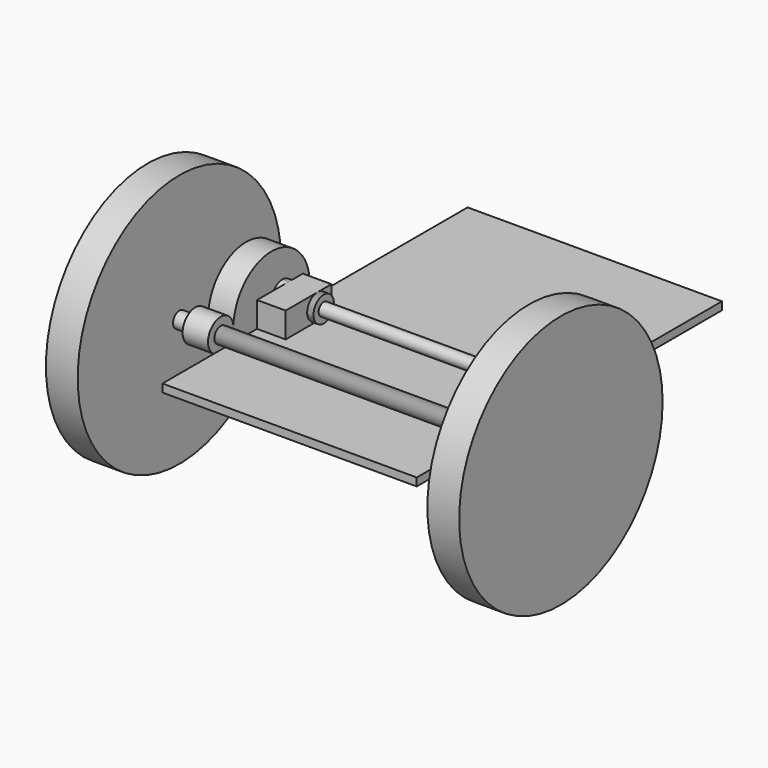
from build123d import *

# Parameters (mm, degrees)
F0_W      = 101.6
F0_H      = 152.4
F1_DEPTH  = 3.175
F3_DEPTH  = 114.3
F4_DEPTH  = 12.7
F5_R      = 6.35
F5_R_2    = 3.175
F6_DEPTH  = 10.16
F7_R      = 3.175
F8_DEPTH  = 6.35
F10_DEPTH = 16.51
F11_W     = 11.43
F11_H     = 22.86
F12_DEPTH = 10.16
F14_DEPTH = 2.54
F15_R     = 2.54
F16_DEPTH = 73.66
F17_DEPTH = 3.81
F18_R     = 5.08
F18_R_2   = 2.54
F19_DEPTH = 2.54
F20_DEPTH = 16.51
F21_DEPTH = 2.54
F22_R     = 50.8
F23_DEPTH = 12.7
F25_DEPTH = 2.54


with BuildPart() as f1:
    # F0 (on Top) → F1 (new body)
    with BuildSketch(Plane.XY):
        Rectangle(F0_W, F0_H)
    extrude(amount=F1_DEPTH)


with BuildPart() as f3:
    # F2 (on face) → F3 (new body)
    with BuildSketch(Plane.YZ.offset(50.8)):
        with BuildLine():
            ThreePointArc((-43.9096465707, 3.175), (-41.6645825404, 4.1049359697), (-40.7346465707, 6.35))
            ThreePointArc((-40.7346465707, 6.35), (-46.1547106009, 8.5950640303), (-43.9096465707, 3.175))
        make_face()
    extrude(amount=-F3_DEPTH)

    # F4 (add): a face of the model
    f4_faces = [f3.faces().sort_by_distance(p)[0] for p in [
        (50.8, -43.9096465707, 6.35),
    ]]
    extrude(f4_faces, amount=F4_DEPTH)

    # F5 (on face) → F6 (join)
    with BuildSketch(Plane.YZ.offset(63.5)):
        with Locations((-43.9096465707, 6.35)):
            Circle(F5_R)
        with Locations((-43.9096465707, 6.35)):
            Circle(F5_R_2, mode=Mode.SUBTRACT)
    extrude(amount=-F6_DEPTH)

    # F7 (on face) → F8 (join)
    with BuildSketch(Plane.YZ.offset(63.5)):
        with Locations((-43.9096465707, 6.35)):
            Circle(F7_R)
    extrude(amount=F8_DEPTH)

    # F22 (on face) → F23 (join)
    with BuildSketch(Plane.YZ.offset(69.85)):
        with Locations((-43.9096465707, 6.35)):
            Circle(F22_R)
    extrude(amount=F23_DEPTH)


with BuildPart() as f10:
    # F9 (on face) → F10 (new body)
    with BuildSketch(Plane.YZ.offset(69.85)):
        with BuildLine():
            ThreePointArc((0.5403534293, 6.35), (-18.5096465707, 25.4), (-37.5596465707, 6.35))
            ThreePointArc((-37.5596465707, 6.35), (-18.5096465707, -12.7), (0.5403534293, 6.35))
        make_face()
    extrude(amount=-F10_DEPTH)

    # F17 (cut): a face of the model
    f17_faces = [f10.faces().sort_by_distance(p)[0] for p in [
        (69.85, -18.5096465707, 6.35),
    ]]
    extrude(f17_faces, amount=-F17_DEPTH, mode=Mode.SUBTRACT)

    # F21 (cut): a face of the model
    f21_faces = [f10.faces().sort_by_distance(p)[0] for p in [
        (66.04, -18.5096465707, 6.35),
    ]]
    extrude(f21_faces, amount=-F21_DEPTH, mode=Mode.SUBTRACT)


with BuildPart() as f12:
    # F11 (on face) → F12 (new body)
    with BuildSketch(Plane.XY.offset(3.175)):
        with Locations((45.085, -17.5209892464)):
            Rectangle(F11_W, F11_H)
    extrude(amount=F12_DEPTH)


with BuildPart() as f14:
    # F13 (on face) → F14 (new body)
    with BuildSketch(Plane(origin=(39.37, 0, 0), x_dir=(0, -1, 0), z_dir=(-1, 0, 0))):
        with BuildLine():
            ThreePointArc((13.1286922842, 3.175), (16.7207947327, 4.6628975516), (18.2086922842, 8.255))
            ThreePointArc((18.2086922842, 8.255), (16.7207947327, 11.8471024484), (13.1286922842, 13.335))
            ThreePointArc((13.1286922842, 13.335), (8.0486922842, 8.255), (13.1286922842, 3.175))
        make_face()
    extrude(amount=F14_DEPTH)


with BuildPart() as f16:
    # F15 (on face) → F16 (new body)
    with BuildSketch(Plane(origin=(36.83, 0, 0), x_dir=(0, -1, 0), z_dir=(-1, 0, 0))):
        with Locations((13.1286922842, 8.255)):
            Circle(F15_R)
    extrude(amount=F16_DEPTH)


with BuildPart() as f19:
    # F18 (on face) → F19 (new body)
    with BuildSketch(Plane(origin=(-36.83, 0, 0), x_dir=(0, -1, 0), z_dir=(-1, 0, 0))):
        with Locations((13.1286922842, 8.255)):
            Circle(F18_R)
        with Locations((13.1286922842, 8.255)):
            Circle(F18_R_2, mode=Mode.SUBTRACT)
    extrude(amount=F19_DEPTH)


with BuildPart() as f20:
    # F20 (new): a face of the model
    f20_faces = [f14.part.faces().sort_by_distance(p)[0] for p in [
        (36.83, -13.1286922842, 8.255),
    ]]
    extrude(f20_faces, amount=-F20_DEPTH)


with BuildPart() as f25:
    # F25 (new): a face of the model
    f25_faces = [f16.part.faces().sort_by_distance(p)[0] for p in [
        (-36.83, -13.1286922842, 8.255),
    ]]
    extrude(f25_faces, amount=F25_DEPTH)


with BuildPart() as f29_1:
    # F29: instance of F3
    add(f3.part.mirror(Plane(origin=(0, 76.2, 3.175), x_dir=(0, -0.9991330731, -0.0416305447), z_dir=(1, 0, 0))))


with BuildPart() as f29_2:
    # F29: instance of F10
    add(f10.part.mirror(Plane(origin=(0, 76.2, 3.175), x_dir=(0, -0.9991330731, -0.0416305447), z_dir=(1, 0, 0))))


with BuildPart() as f29_3:
    # F29: instance of F12
    add(f12.part.mirror(Plane(origin=(0, 76.2, 3.175), x_dir=(0, -0.9991330731, -0.0416305447), z_dir=(1, 0, 0))))


with BuildPart() as f29_4:
    # F29: instance of F14
    add(f14.part.mirror(Plane(origin=(0, 76.2, 3.175), x_dir=(0, -0.9991330731, -0.0416305447), z_dir=(1, 0, 0))))


with BuildPart() as f29_5:
    # F29: instance of F16
    add(f16.part.mirror(Plane(origin=(0, 76.2, 3.175), x_dir=(0, -0.9991330731, -0.0416305447), z_dir=(1, 0, 0))))


with BuildPart() as f29_6:
    # F29: instance of F20
    add(f20.part.mirror(Plane(origin=(0, 76.2, 3.175), x_dir=(0, -0.9991330731, -0.0416305447), z_dir=(1, 0, 0))))


with BuildPart() as f29_7:
    # F29: instance of F19
    add(f19.part.mirror(Plane(origin=(0, 76.2, 3.175), x_dir=(0, -0.9991330731, -0.0416305447), z_dir=(1, 0, 0))))


solid = Compound([f1.part, f3.part, f10.part, f12.part, f14.part, f16.part, f19.part, f20.part, f25.part, f29_1.part, f29_2.part, f29_3.part, f29_4.part, f29_5.part, f29_6.part, f29_7.part])
